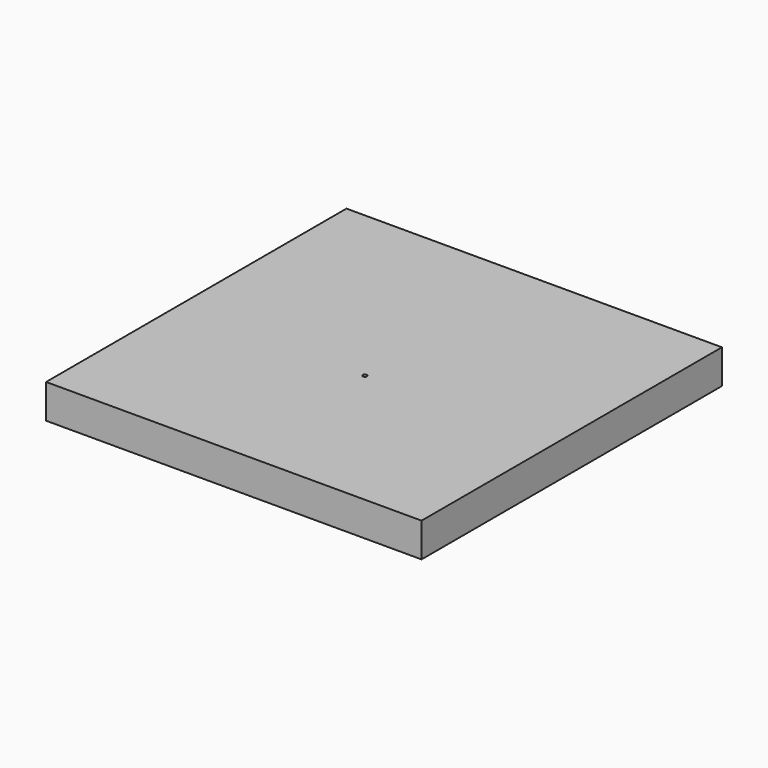
from build123d import *

# Parameters (mm, degrees)
F0_W     = 550
F0_H     = 550
F0_R     = 3
F0_W_2   = 50
F0_H_2   = 50
F1_DEPTH = 50


with BuildPart() as f1:
    # F0 (on Top) → F1 (new body)
    with BuildSketch(Plane.XY):
        Rectangle(F0_W, F0_H)
        Polygon((222.5, 272.5), (272.5, 272.5), (272.5, 222.5), (272.5, -222.5), (272.5, -272.5), (222.5, -272.5), (-222.5, -272.5), (-272.5, -272.5), (-272.5, -222.5), (-272.5, 222.5), (-272.5, 272.5), (-222.5, 272.5), align=None, mode=Mode.SUBTRACT)
        Polygon((222.5, 222.5), (222.5, 272.5), (-222.5, 272.5), (-222.5, 222.5), (-272.5, 222.5), (-272.5, -222.5), (-222.5, -222.5), (-222.5, -272.5), (222.5, -272.5), (222.5, -222.5), (272.5, -222.5), (272.5, 222.5), align=None)
        with Locations((0, -35)):
            Circle(F0_R, mode=Mode.SUBTRACT)
        with Locations((-247.5, 247.5)):
            Rectangle(F0_W_2, F0_H_2)
        with Locations((247.5, -247.5)):
            Rectangle(F0_W_2, F0_H_2)
        with Locations((247.5, 247.5)):
            Rectangle(F0_W_2, F0_H_2)
        with Locations((-247.5, -247.5)):
            Rectangle(F0_W_2, F0_H_2)
    extrude(amount=F1_DEPTH)


solid = f1.part
